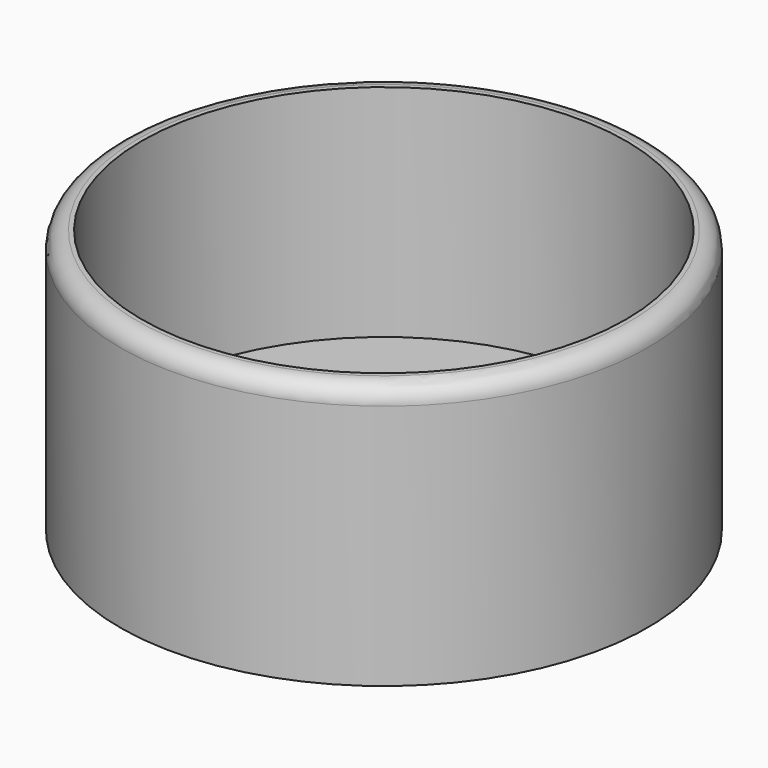
from build123d import *

# Parameters (mm, degrees)
F0_W     = 76.2
F0_H     = 76.2
F2_R     = 69.8500005424
F3_DEPTH = 63.5
F4_R     = 5.08


with BuildPart() as f1:
    # F0 (on Front) → F1 (revolve)
    with BuildSketch(Plane.XZ):
        Rectangle(F0_W, F0_H)
    revolve(axis=Axis((38.1, 0, 0), (0, 0, -1)))

    # F2 (on face) → F3 (cut)
    with BuildSketch(Plane.XY.offset(38.1)):
        with Locations((38.1, 0)):
            Circle(F2_R)
    extrude(amount=-F3_DEPTH, mode=Mode.SUBTRACT)

    # F4
    f4_edges = [f1.edges().sort_by_distance(p)[0] for p in [
        (114.3, 0, 38.1),
    ]]
    fillet(f4_edges, radius=F4_R)


solid = f1.part
